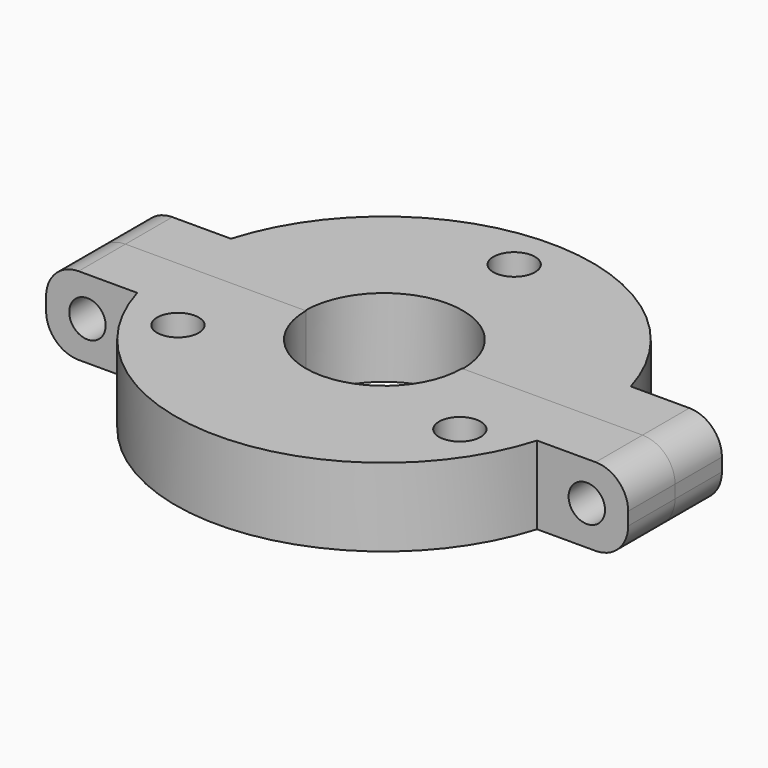
from build123d import *

# Parameters (mm, degrees)
F0_R      = 1.6
F1_DEPTH  = 3
F2_DEPTH  = 3
F3_R      = 1.4
F4_DEPTH  = 16.001
F5_R      = 2.5
F6_R      = 1.6
F7_DEPTH  = 3
F8_DEPTH  = 3
F9_R      = 1.4
F10_DEPTH = 25
F11_R     = 2.5


# Not quite as in the source:
# - a feature names something its author has since deleted; it is built from what else it names


with BuildPart() as f1:
    # F0 (on Top) → F1 (new body)
    with BuildSketch(Plane.XY):
        with BuildLine():
            ThreePointArc((-16, 0), (-15.8377151213, 2.273055155), (-15.3541525328, 4.5))
            Line((-15.3541525328, 4.5), (-22.3541525328, 4.5))
            Line((-22.3541525328, 4.5), (-22.3541525328, 0))
            Line((-22.3541525328, 0), (-16, 0))
        make_face()
        with BuildLine():
            Line((7.65, 0), (16, 0))
            ThreePointArc((16, 0), (15.8377151213, 2.273055155), (15.3541525328, 4.5))
            ThreePointArc((15.3541525328, 4.5), (0, 16), (-15.3541525328, 4.5))
            ThreePointArc((-15.3541525328, 4.5), (-15.8377151213, 2.273055155), (-16, 0))
            Line((-16, 0), (-7.65, 0))
            ThreePointArc((-7.65, 0), (0, 7.65), (7.65, 0))
        make_face()
        with Locations((0, 12.5)):
            Circle(F0_R, mode=Mode.SUBTRACT)
        with BuildLine():
            ThreePointArc((-6.05, 0), (0, 6.05), (6.05, 0))
            Line((6.05, 0), (7.65, 0))
            ThreePointArc((7.65, 0), (0, 7.65), (-7.65, 0))
            Line((-7.65, 0), (-6.05, 0))
        make_face()
        with BuildLine():
            ThreePointArc((15.3541525328, 4.5), (15.8377151213, 2.273055155), (16, 0))
            Line((16, 0), (22.3541525328, 0))
            Line((22.3541525328, 0), (22.3541525328, 4.5))
            Line((22.3541525328, 4.5), (15.3541525328, 4.5))
        make_face()
    extrude(amount=F1_DEPTH)

    # F0 (on Top) → F2 (join)
    with BuildSketch(Plane.XY):
        with BuildLine():
            Line((7.65, 0), (16, 0))
            ThreePointArc((16, 0), (15.8377151213, 2.273055155), (15.3541525328, 4.5))
            ThreePointArc((15.3541525328, 4.5), (0, 16), (-15.3541525328, 4.5))
            ThreePointArc((-15.3541525328, 4.5), (-15.8377151213, 2.273055155), (-16, 0))
            Line((-16, 0), (-7.65, 0))
            ThreePointArc((-7.65, 0), (0, 7.65), (7.65, 0))
        make_face()
        with Locations((0, 12.5)):
            Circle(F0_R, mode=Mode.SUBTRACT)
        with BuildLine():
            ThreePointArc((-6.05, 0), (0, 6.05), (6.05, 0))
            Line((6.05, 0), (7.65, 0))
            ThreePointArc((7.65, 0), (0, 7.65), (-7.65, 0))
            Line((-7.65, 0), (-6.05, 0))
        make_face()
        with BuildLine():
            ThreePointArc((15.3541525328, 4.5), (15.8377151213, 2.273055155), (16, 0))
            Line((16, 0), (22.3541525328, 0))
            Line((22.3541525328, 0), (22.3541525328, 4.5))
            Line((22.3541525328, 4.5), (15.3541525328, 4.5))
        make_face()
        with BuildLine():
            ThreePointArc((-16, 0), (-15.8377151213, 2.273055155), (-15.3541525328, 4.5))
            Line((-15.3541525328, 4.5), (-22.3541525328, 4.5))
            Line((-22.3541525328, 4.5), (-22.3541525328, 0))
            Line((-22.3541525328, 0), (-16, 0))
        make_face()
    extrude(amount=-F2_DEPTH)

    # F3 (on face) → F4 (cut, through all)
    with BuildSketch(Plane.XZ):
        with Locations((19.1770762664, 0)):
            Circle(F3_R)
        with Locations((-19.1770762664, 0)):
            Circle(F3_R)
    extrude(amount=-F4_DEPTH, mode=Mode.SUBTRACT)

    # F5
    f5_edges = [f1.edges().sort_by_distance(p)[0] for p in [
        (-22.354153, 2.25, 3),
        (22.354153, 2.25, 3),
        (-22.354153, 2.25, -3),
        (22.354153, 2.25, -3),
    ]]
    fillet(f5_edges, radius=F5_R)


with BuildPart() as f7:
    # F6 (on Top) → F7 (new body)
    with BuildSketch(Plane.XY):
        with BuildLine():
            ThreePointArc((6, 0), (0, -6), (-6, 0))
            Line((-6, 0), (-9, 0))
            ThreePointArc((-9, 0), (0, -9), (9, 0))
            Line((9, 0), (6, 0))
        make_face()
        with BuildLine():
            ThreePointArc((9, 0), (0, -9), (-9, 0))
            Line((-9, 0), (-16, 0))
            ThreePointArc((-16, 0), (-15.8377151213, -2.273055155), (-15.3541525328, -4.5))
            ThreePointArc((-15.3541525328, -4.5), (0, -16), (15.3541525328, -4.5))
            ThreePointArc((15.3541525328, -4.5), (15.8377151213, -2.273055155), (16, 0))
            Line((16, 0), (9, 0))
        make_face()
        with Locations((-10.8253175473, -6.25)):
            Circle(F6_R, mode=Mode.SUBTRACT)
        with Locations((10.8253175473, -6.25)):
            Circle(F6_R, mode=Mode.SUBTRACT)
        with BuildLine():
            ThreePointArc((-15.3541525328, -4.5), (-15.8377151213, -2.273055155), (-16, 0))
            Line((-16, 0), (-22.3541525328, 0))
            Line((-22.3541525328, 0), (-22.3541525328, -4.5))
            Line((-22.3541525328, -4.5), (-15.3541525328, -4.5))
        make_face()
        with BuildLine():
            Line((22.3541525328, 0), (16, 0))
            ThreePointArc((16, 0), (15.8377151213, -2.273055155), (15.3541525328, -4.5))
            Line((15.3541525328, -4.5), (22.3541525328, -4.5))
            Line((22.3541525328, -4.5), (22.3541525328, 0))
        make_face()
    extrude(amount=-F7_DEPTH)

    # F6 (on Top) → F8 (join)
    with BuildSketch(Plane.XY):
        with BuildLine():
            ThreePointArc((-15.3541525328, -4.5), (-15.8377151213, -2.273055155), (-16, 0))
            Line((-16, 0), (-22.3541525328, 0))
            Line((-22.3541525328, 0), (-22.3541525328, -4.5))
            Line((-22.3541525328, -4.5), (-15.3541525328, -4.5))
        make_face()
        with BuildLine():
            Line((22.3541525328, 0), (16, 0))
            ThreePointArc((16, 0), (15.8377151213, -2.273055155), (15.3541525328, -4.5))
            Line((15.3541525328, -4.5), (22.3541525328, -4.5))
            Line((22.3541525328, -4.5), (22.3541525328, 0))
        make_face()
        with BuildLine():
            ThreePointArc((9, 0), (0, -9), (-9, 0))
            Line((-9, 0), (-16, 0))
            ThreePointArc((-16, 0), (-15.8377151213, -2.273055155), (-15.3541525328, -4.5))
            ThreePointArc((-15.3541525328, -4.5), (0, -16), (15.3541525328, -4.5))
            ThreePointArc((15.3541525328, -4.5), (15.8377151213, -2.273055155), (16, 0))
            Line((16, 0), (9, 0))
        make_face()
        with Locations((-10.8253175473, -6.25)):
            Circle(F6_R, mode=Mode.SUBTRACT)
        with Locations((10.8253175473, -6.25)):
            Circle(F6_R, mode=Mode.SUBTRACT)
        with BuildLine():
            ThreePointArc((6, 0), (0, -6), (-6, 0))
            Line((-6, 0), (-9, 0))
            ThreePointArc((-9, 0), (0, -9), (9, 0))
            Line((9, 0), (6, 0))
        make_face()
    extrude(amount=F8_DEPTH)

    # F9 (on face) → F10 (cut)
    with BuildSketch(Plane.XZ.offset(4.5)):
        with Locations((-19.1770762664, 0)):
            Circle(F9_R)
        with Locations((19.1770762664, 0)):
            Circle(F9_R)
    extrude(amount=-F10_DEPTH, mode=Mode.SUBTRACT)

    # F11
    f11_edges = [f7.edges().sort_by_distance(p)[0] for p in [
        (22.354153, -2.25, -3),
        (22.354153, -2.25, 3),
        (-22.354153, -2.25, 3),
        (-22.354153, -2.25, -3),
    ]]
    fillet(f11_edges, radius=F11_R)


solid = Compound([f1.part, f7.part])
